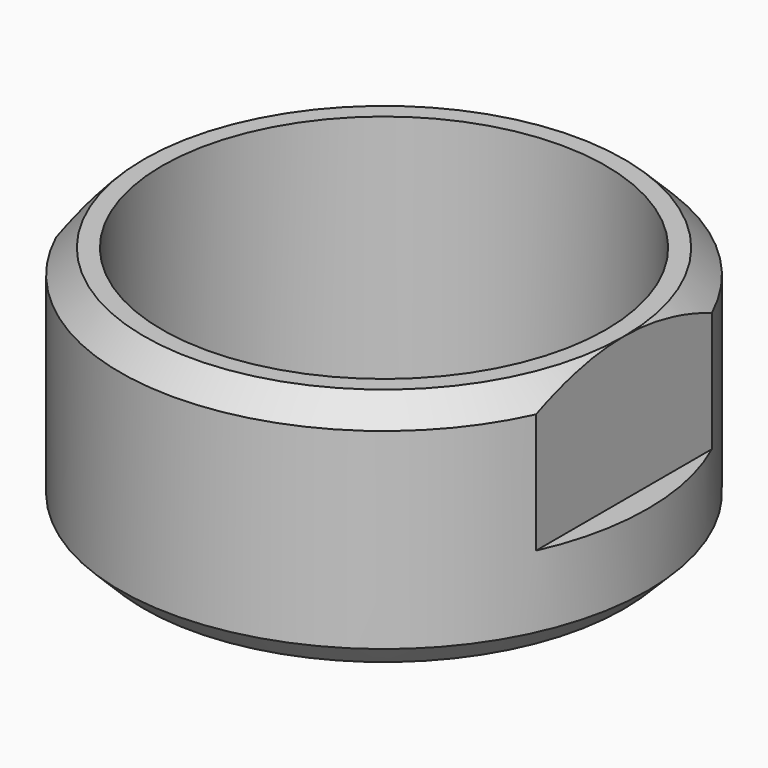
from build123d import *

# Parameters (mm, degrees)
F0_R     = 11
F0_R_2   = 9.25
F1_DEPTH = 10
F3_DEPTH = 6
F4_SIZE  = 0.99999


# Not quite as in the source:
# - a fillet or chamfer is up to 0.001 mm smaller than in the source, because OpenCascade refuses the exact size


with BuildPart() as f1:
    # F0 (on Top) → F1 (new body)
    with BuildSketch(Plane.XY):
        Circle(F0_R)
        Circle(F0_R_2, mode=Mode.SUBTRACT)
    extrude(amount=F1_DEPTH)

    # F2 (on face) → F3 (cut)
    with BuildSketch(Plane.XY.offset(10)):
        with BuildLine():
            Line((-10, -4.582575695), (-10, 4.582575695))
            ThreePointArc((-10, 4.582575695), (-11, 0), (-10, -4.582575695))
        make_face()
        with BuildLine():
            ThreePointArc((11, 0), (10.7470926301, 2.3452078799), (10, 4.582575695))
            Line((10, 4.582575695), (10, -4.582575695))
            ThreePointArc((10, -4.582575695), (10.7470926301, -2.3452078799), (11, 0))
        make_face()
    extrude(amount=-F3_DEPTH, mode=Mode.SUBTRACT)

    # F4 (size 1 in the source; OpenCascade refuses exactly that, so slightly less here)
    f4_edges = [f1.edges().sort_by_distance(p)[0] for p in [
        (-11, 0, 0),
        (0, -11, 10),
        (0, 11, 10),
    ]]
    chamfer(f4_edges, length=F4_SIZE)


solid = f1.part
